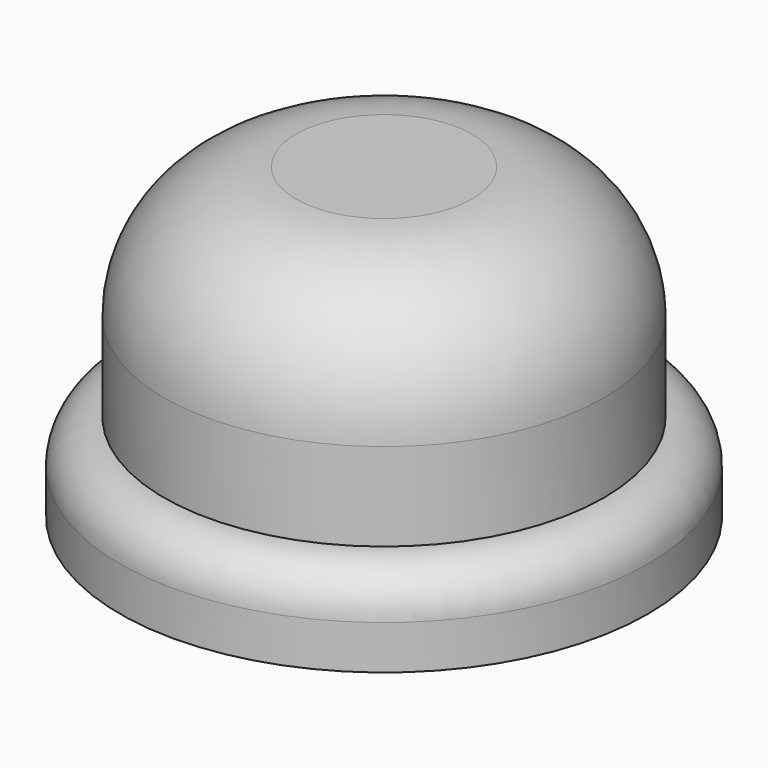
from build123d import *

# Parameters (mm, degrees)
F0_R     = 5
F1_DEPTH = 5
F2_R     = 3
F3_R     = 6
F3_R_2   = 5
F4_DEPTH = 2
F5_R     = 0.99999
F6_R     = 1.75
F7_DEPTH = 4


# Not quite as in the source:
# - a fillet or chamfer is up to 0.001 mm smaller than in the source, because OpenCascade refuses the exact size


with BuildPart() as f1:
    # F0 (on Top) → F1 (new body)
    with BuildSketch(Plane.XY):
        Circle(F0_R)
    extrude(amount=F1_DEPTH)

    # F2
    f2_edges = [f1.edges().sort_by_distance(p)[0] for p in [
        (-5, 0, 5),
    ]]
    fillet(f2_edges, radius=F2_R)

    # F3 (on face) → F4 (join)
    with BuildSketch(Plane(origin=(0, 0, 0), x_dir=(1, 0, 0), z_dir=(0, 0, -1))):
        Circle(F3_R)
        Circle(F3_R_2, mode=Mode.SUBTRACT)
        Circle(F3_R_2)
    extrude(amount=F4_DEPTH)

    # F5 (radius 1 in the source; OpenCascade refuses exactly that, so slightly less here)
    f5_edges = [f1.edges().sort_by_distance(p)[0] for p in [
        (-6, 0, 0),
    ]]
    fillet(f5_edges, radius=F5_R)

    # F6 (on face) → F7 (cut)
    with BuildSketch(Plane(origin=(0, 0, -2), x_dir=(1, 0, 0), z_dir=(0, 0, -1))):
        Circle(F6_R)
    extrude(amount=-F7_DEPTH, mode=Mode.SUBTRACT)


solid = f1.part
